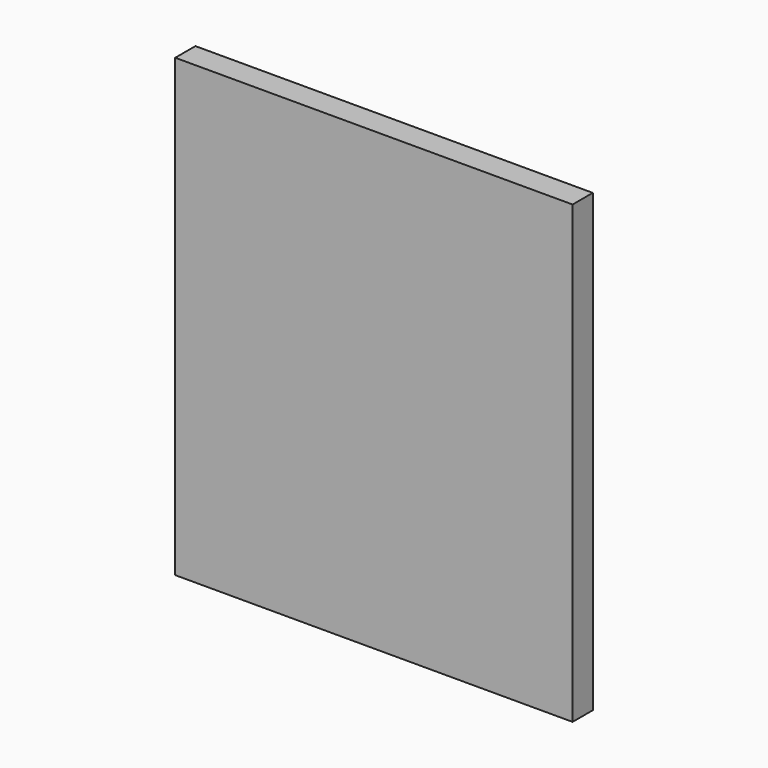
from build123d import *

# Parameters (mm, degrees)
F1_DEPTH = 6.35


# Not quite as in the source:
# - a feature names something its author has since deleted; it is built from what else it names


with BuildPart() as f1:
    # F0 (on Front) → F1 (new body)
    with BuildSketch(Plane.XZ):
        Polygon((-50, -50), (50, -50), (50, 50), (50, 64.6395087242), (-50, 64.6395087242), (-50, 50), align=None)
    extrude(amount=F1_DEPTH)


solid = f1.part
